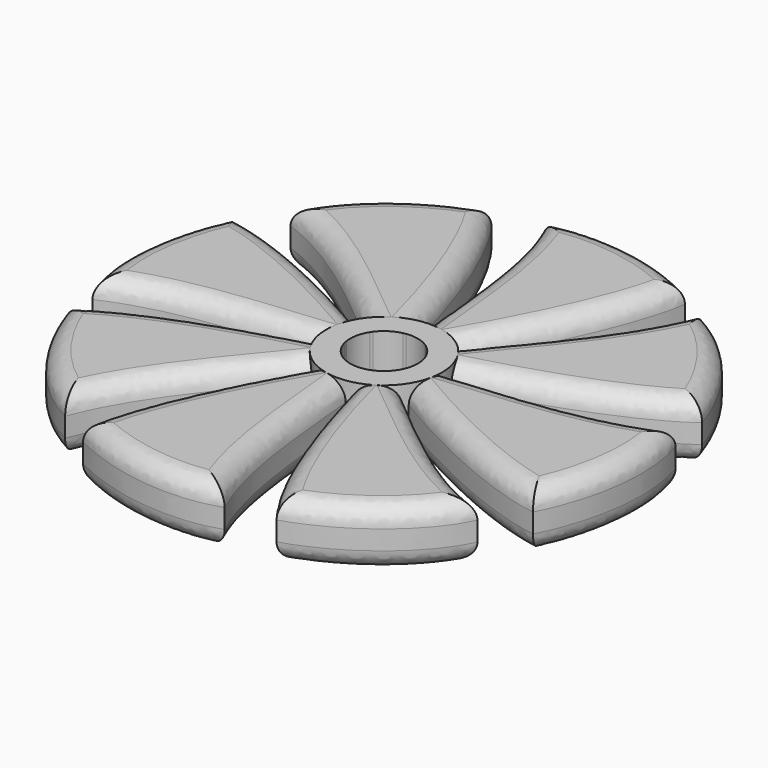
from build123d import *

# Parameters (mm, degrees)
F1_DEPTH = 3
F2_COUNT = 8
F3_DEPTH = 3
F4_R     = 1
F5_R     = 1


with BuildPart() as f1:
    # F0 (on Top) → F1 (new body)
    with BuildSketch(Plane.XY):
        with BuildLine():
            add(Edge.make_bspline(
                [(1.8216950039, 2.3835744824), (4.0666955785, 5.1494965145), (6.530272224, 7.8355872147), (7.6986034113, 10.9947451166)],
                knots=[2.9640247987, 2.9640247987, 2.9640247987, 2.9640247987, 13.4221054482, 13.4221054482, 13.4221054482, 13.4221054482], degree=3))
            ThreePointArc((1.8216950039, 2.3835744824), (2.5200827694, 1.6276310502), (2.9218859296, 0.6801342618))
            add(Edge.make_bspline(
                [(2.9218859296, 0.6801342618), (6.7951188387, 1.6840982203), (10.7030554056, 3.1088325628), (12.7462048342, 4.6392391595)],
                knots=[2.75386921, 2.75386921, 2.75386921, 2.75386921, 13.564227868, 13.564227868, 13.564227868, 13.564227868], degree=3))
            add(Edge.make_bspline(
                [(7.6986034113, 10.9947451166), (9.8994949366, 9.8994949366), (11.8474765443, 7.459041462), (12.7462048342, 4.6392391595)],
                knots=[0, 0, 0, 0, 8.116078862, 8.116078862, 8.116078862, 8.116078862], degree=3))
        make_face()
        with BuildLine():
            ThreePointArc((2.9218859296, 0.6801342618), (2.5200827694, 1.6276310502), (1.8216950039, 2.3835744824))
            add(Edge.make_bspline(
                [(1.0426793893, 1.4054606687), (1.297708333, 1.73319436), (1.5581961111, 2.0589343013), (1.8216950039, 2.3835744824)],
                knots=[1.736545081, 1.736545081, 1.736545081, 1.736545081, 2.9640247987, 2.9640247987, 2.9640247987, 2.9640247987], degree=3))
            ThreePointArc((1.0426793893, 1.4054606687), (1.4682114829, 0.9522893686), (1.7084772015, 0.3789533638))
            add(Edge.make_bspline(
                [(1.7084772015, 0.3789533638), (2.1111123241, 0.4744921588), (2.516308868, 0.575006385), (2.9218859296, 0.6801342618)],
                knots=[1.6218862897, 1.6218862897, 1.6218862897, 1.6218862897, 2.75386921, 2.75386921, 2.75386921, 2.75386921], degree=3))
        make_face()
    extrude(amount=F1_DEPTH)


with BuildPart() as f2_1:
    # F2: instance of F1
    add(f1.part.rotate(Axis((0, 0, 0), (0, 0, 1)), 1 * 360 / F2_COUNT))


with BuildPart() as f2_2:
    # F2: instance of F1
    add(f1.part.rotate(Axis((0, 0, 0), (0, 0, 1)), 2 * 360 / F2_COUNT))


with BuildPart() as f2_3:
    # F2: instance of F1
    add(f1.part.rotate(Axis((0, 0, 0), (0, 0, 1)), 3 * 360 / F2_COUNT))


with BuildPart() as f2_4:
    # F2: instance of F1
    add(f1.part.rotate(Axis((0, 0, 0), (0, 0, 1)), 4 * 360 / F2_COUNT))


with BuildPart() as f2_5:
    # F2: instance of F1
    add(f1.part.rotate(Axis((0, 0, 0), (0, 0, 1)), 5 * 360 / F2_COUNT))


with BuildPart() as f2_6:
    # F2: instance of F1
    add(f1.part.rotate(Axis((0, 0, 0), (0, 0, 1)), 6 * 360 / F2_COUNT))


with BuildPart() as f2_7:
    # F2: instance of F1
    add(f1.part.rotate(Axis((0, 0, 0), (0, 0, 1)), 7 * 360 / F2_COUNT))


with BuildPart() as f1_1:
    add(f1.part)

    add(f2_1.part)  # F3 merges F2_1

    add(f2_2.part)  # F3 merges F2_2

    add(f2_3.part)  # F3 merges F2_3

    add(f2_4.part)  # F3 merges F2_4

    add(f2_5.part)  # F3 merges F2_5

    add(f2_6.part)  # F3 merges F2_6

    add(f2_7.part)  # F3 merges F2_7
    # F0 (on Top) → F3 (join)
    with BuildSketch(Plane.XY):
        with BuildLine():
            Line((1.2374368671, -1.2374368671), (2.1213203436, -2.1213203436))
            ThreePointArc((2.1213203436, -2.1213203436), (2.7716385975, -1.1480502971), (3, 0))
            ThreePointArc((3, 0), (2.9804075048, 0.3423026519), (2.9218859296, 0.6801342618))
            add(Edge.make_bspline(
                [(1.7084772015, 0.3789533638), (2.1111123241, 0.4744921588), (2.516308868, 0.575006385), (2.9218859296, 0.6801342618)],
                knots=[1.6218862897, 1.6218862897, 1.6218862897, 1.6218862897, 2.75386921, 2.75386921, 2.75386921, 2.75386921], degree=3))
            ThreePointArc((1.7084772015, 0.3789533638), (1.7395883281, 0.1906107255), (1.75, 0))
            ThreePointArc((1.75, 0), (1.6167891819, -0.6696960066), (1.2374368671, -1.2374368671))
        make_face()
        with BuildLine():
            ThreePointArc((1.8216950039, 2.3835744824), (-2.9933863525, -0.1990933057), (2.1213203436, -2.1213203436))
            Line((2.1213203436, -2.1213203436), (1.2374368671, -1.2374368671))
            ThreePointArc((1.2374368671, -1.2374368671), (-1.7452677106, -0.128610335), (1.0426793893, 1.4054606687))
            add(Edge.make_bspline(
                [(1.0426793893, 1.4054606687), (1.297708333, 1.73319436), (1.5581961111, 2.0589343013), (1.8216950039, 2.3835744824)],
                knots=[1.736545081, 1.736545081, 1.736545081, 1.736545081, 2.9640247987, 2.9640247987, 2.9640247987, 2.9640247987], degree=3))
        make_face()
    extrude(amount=F3_DEPTH)

    # F4
    f4_edges = [f1_1.edges().sort_by_distance(p)[0] for p in [
        (-13.534561, 1.782793, 3),
        (-8.180973, -0.959915, 3),
        (-7.258125, 4.057309, 3),
        (-6.463584, 5.106059, 3),
        (-8.309754, 10.831005, 3),
        (-2.263319, 8.00122, 3),
        (-0.959915, 8.180973, 3),
        (1.782793, 13.534561, 3),
        (4.057309, 7.258125, 3),
        (5.106059, 6.463584, 3),
        (10.831005, 8.309754, 3),
        (8.00122, 2.263319, 3),
        (8.180973, 0.959915, 3),
        (13.534561, -1.782793, 3),
        (7.258125, -4.057309, 3),
        (6.463584, -5.106059, 3),
        (2.263319, -8.00122, 3),
        (0.959915, -8.180973, 3),
        (-4.057309, -7.258125, 3),
        (-5.106059, -6.463584, 3),
        (-8.00122, -2.263319, 3),
        (-10.831005, -8.309754, 3),
        (-1.782793, -13.534561, 3),
        (8.309754, -10.831005, 3),
    ]]
    fillet(f4_edges, radius=F4_R)

    # F5
    f5_edges = [f1_1.edges().sort_by_distance(p)[0] for p in [
        (5.106059, 6.463584, 0),
        (10.831005, 8.309754, 0),
        (8.00122, 2.263319, 0),
        (4.057309, 7.258125, 0),
        (1.782793, 13.534561, 0),
        (-0.959915, 8.180973, 0),
        (-2.263319, 8.00122, 0),
        (-8.309754, 10.831005, 0),
        (-6.463584, 5.106059, 0),
        (-7.258125, 4.057309, 0),
        (-13.534561, 1.782793, 0),
        (-8.180973, -0.959915, 0),
        (-8.00122, -2.263319, 0),
        (-10.831005, -8.309754, 0),
        (-5.106059, -6.463584, 0),
        (-4.057309, -7.258125, 0),
        (0.959915, -8.180973, 0),
        (8.180973, 0.959915, 0),
        (13.534561, -1.782793, 0),
        (7.258125, -4.057309, 0),
        (6.463584, -5.106059, 0),
        (2.263319, -8.00122, 0),
        (-1.782793, -13.534561, 0),
        (8.309754, -10.831005, 0),
    ]]
    fillet(f5_edges, radius=F5_R)


solid = f1_1.part
